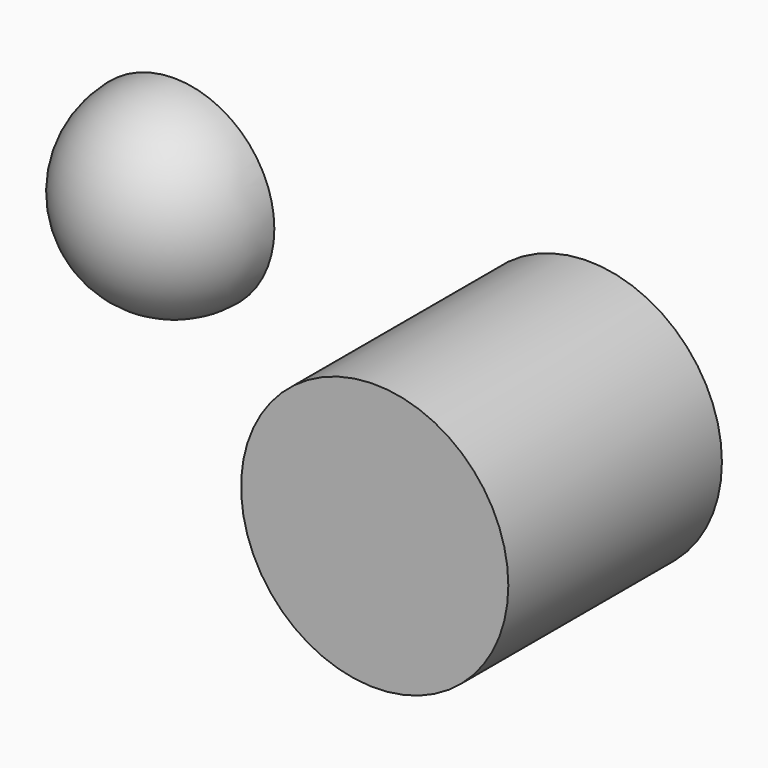
from build123d import *

# Parameters (mm, degrees)
F0_R     = 40.0379704722
F1_DEPTH = 80
F7_ANGLE = 180


# Not quite as in the source:
# - the program builds the solid bodies; features that only make, move or delete a surface that nothing else refers to are left out


with BuildPart() as f1:
    # F0 (on Front) → F1 (new body)
    with BuildSketch(Plane.XZ):
        Circle(F0_R)
    extrude(amount=F1_DEPTH)

    # F2 (on Front) → F3 (revolve, cut)
    with BuildSketch(Plane.XZ):
        with BuildLine():
            Line((0, 20.2877700597), (0, -19.7122299403))
            ThreePointArc((0, -19.7122299403), (20, 0.2877700597), (0, 20.2877700597))
        make_face()
    revolve(axis=Axis((0, 0, 0.2877700597), (0, 0, 1)), mode=Mode.SUBTRACT)


with BuildPart() as f7:
    # F6 (on Front) → F7 (revolve)
    with BuildSketch(Plane.XZ):
        with BuildLine():
            ThreePointArc((-124.0761767042, 47.9414828308), (-154.0761767042, 17.9414828308), (-124.0761767042, -12.0585171692))
            Line((-124.0761767042, -12.0585171692), (-124.0761767042, 47.9414828308))
        make_face()
    revolve(axis=Axis((-124.0761767042, 0, 17.9414828308), (0, 0, 1)), revolution_arc=F7_ANGLE)


solid = Compound([f1.part, f7.part])
